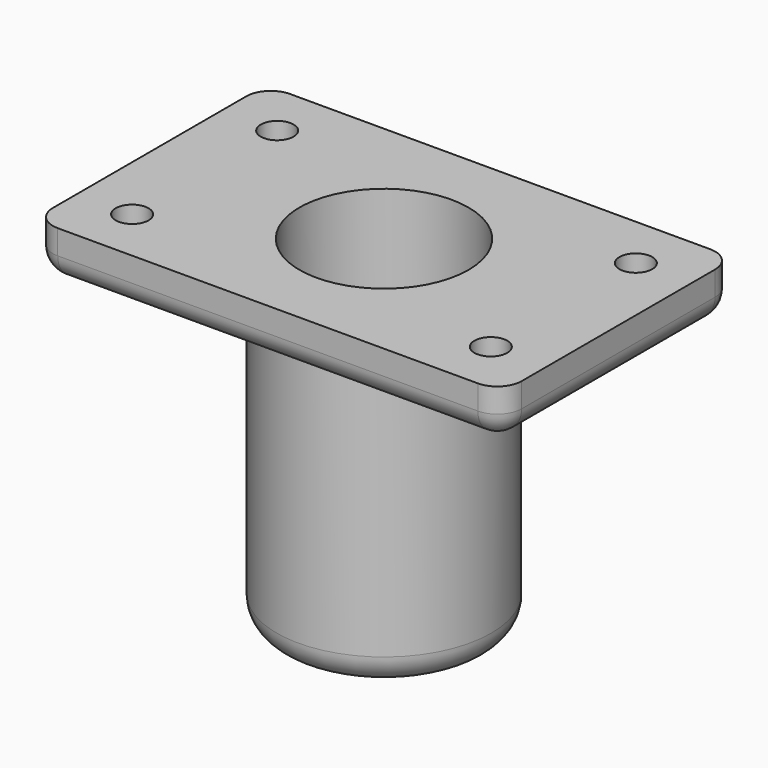
from build123d import *

# Parameters (mm, degrees)
F0_R     = 27.9704951592
F0_R_2   = 22.0413133634
F1_DEPTH = 76.2
F3_DEPTH = 12.7
F5_R     = 6.35
F6_R     = 4.2845599963
F7_DEPTH = 25.4
F8_DEPTH = 25.4


# Not quite as in the source:
# - a fillet or chamfer that OpenCascade refuses, or shapes differently, is made with other operations: its cross-section is extruded or revolved along the edge and cut away or added


with BuildPart() as f1:
    # F0 (on Top) → F1 (new body)
    with BuildSketch(Plane.XY):
        Circle(F0_R)
        Circle(F0_R_2, mode=Mode.SUBTRACT)
    extrude(amount=F1_DEPTH)

    # F2 (on face) → F3 (join)
    with BuildSketch(Plane.XY.offset(76.2)):
        with BuildLine():
            Line((-54.7763327301, -37.8764942288), (54.7763327301, -37.8764942288))
            ThreePointArc((54.7763327301, -37.8764942288), (59.2664607906, -36.0166222894), (61.1263327301, -31.5264942288))
            Line((61.1263327301, -31.5264942288), (61.1263327301, 31.5264942288))
            ThreePointArc((61.1263327301, 31.5264942288), (59.2664607906, 36.0166222894), (54.7763327301, 37.8764942288))
            Line((54.7763327301, 37.8764942288), (-54.7763327301, 37.8764942288))
            ThreePointArc((-54.7763327301, 37.8764942288), (-59.2664607906, 36.0166222894), (-61.1263327301, 31.5264942288))
            Line((-61.1263327301, 31.5264942288), (-61.1263327301, -31.5264942288))
            ThreePointArc((-61.1263327301, -31.5264942288), (-59.2664607906, -36.0166222894), (-54.7763327301, -37.8764942288))
        make_face()
    extrude(amount=F3_DEPTH)

    # F4: fillet of radius 7.62 on 1 edges, made by hand

    # F4_s1 → F4_t2 (revolve, cut)
    with BuildSketch(Plane.XZ):
        with BuildLine():
            ThreePointArc((27.9704951592, 7.4300426513), (26.3065187789, 2.6771295823), (22.0413133634, 0))
            Line((22.0413133634, 0), (27.9704951592, 0))
            Line((27.9704951592, 0), (27.9704951592, 7.4300426513))
        make_face()
    revolve(axis=Axis((0, 0, 0), (0, 0, 1)), mode=Mode.SUBTRACT)

    # F5
    f5_edges = [f1.edges().sort_by_distance(p)[0] for p in [
        (-61.126333, 0, 76.2),
        (0, -37.876494, 76.2),
        (61.126333, 0, 76.2),
        (0, 37.876494, 76.2),
        (-59.266461, -36.016622, 76.2),
        (59.266461, -36.016622, 76.2),
        (-59.266461, 36.016622, 76.2),
        (59.266461, 36.016622, 76.2),
    ]]
    fillet(f5_edges, radius=F5_R)

    # F6 (on face) → F7 (cut)
    with BuildSketch(Plane(origin=(0, 0, 76.2), x_dir=(1, 0, 0), z_dir=(0, 0, -1))):
        with Locations((46.7646792531, -23.6378517002)):
            Circle(F6_R)
        with Locations((-46.7646792531, -23.6378517002)):
            Circle(F6_R)
        with Locations((46.7646792531, 23.6378517002)):
            Circle(F6_R)
        with Locations((-46.7646792531, 23.6378517002)):
            Circle(F6_R)
    extrude(amount=-F7_DEPTH, mode=Mode.SUBTRACT)

    # F8 (cut): a face of the model
    f8_faces = [f1.faces().sort_by_distance(p)[0] for p in [
        (0, 0, 76.2),
    ]]
    extrude(f8_faces, amount=-F8_DEPTH, mode=Mode.SUBTRACT)


solid = f1.part
